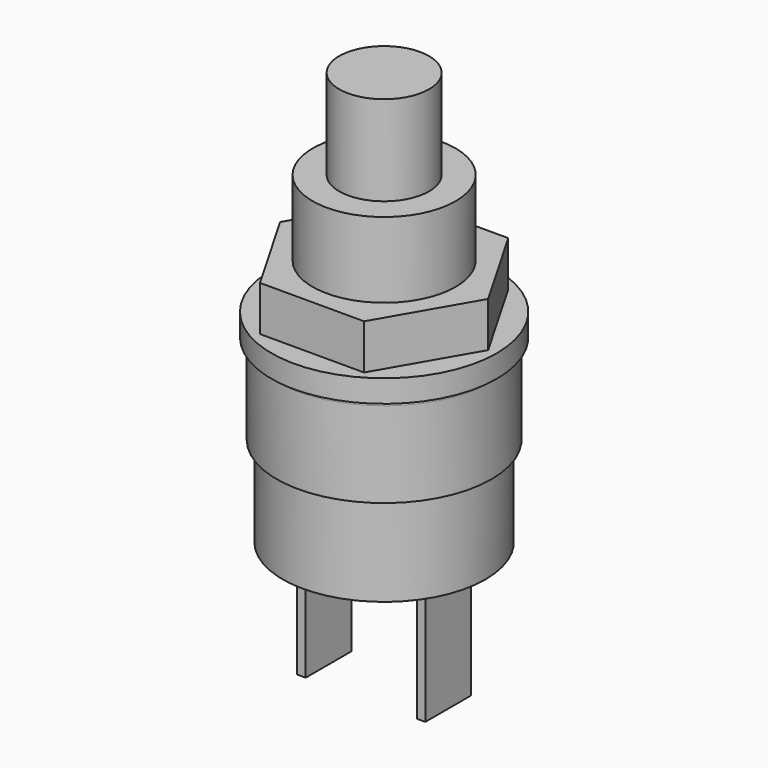
from build123d import *

# Parameters (mm, degrees)
F0_R      = 1.995
F1_DEPTH  = 14.34
F0_R_2    = 3.175
F2_DEPTH  = 10.35
F0_R_3    = 4.765
F0_R_4    = 4.5
F3_DEPTH  = 4
F4_DEPTH  = 4
F5_W      = 0.38
F5_H      = 2.54
F6_DEPTH  = 5.59
F7_R      = 0.2
F8_R      = 5
F8_R_2    = 3.4
F9_DEPTH  = 1
F10_R     = 2.75
F11_DEPTH = 2


with BuildPart() as f1:
    # F0 (on Top) → F1 (new body)
    with BuildSketch(Plane.XY):
        Circle(F0_R)
    extrude(amount=F1_DEPTH)


with BuildPart() as f2:
    # F0 (on Top) → F2 (new body)
    with BuildSketch(Plane.XY):
        Circle(F0_R_2)
        Circle(F0_R, mode=Mode.SUBTRACT)
        Circle(F0_R)
    extrude(amount=F2_DEPTH)

    # F0 (on Top) → F3 (join)
    with BuildSketch(Plane.XY):
        Circle(F0_R_3)
        Circle(F0_R_4, mode=Mode.SUBTRACT)
        Circle(F0_R_4)
        Circle(F0_R_2, mode=Mode.SUBTRACT)
        Circle(F0_R_2)
        Circle(F0_R, mode=Mode.SUBTRACT)
        Circle(F0_R)
    extrude(amount=F3_DEPTH)

    # F0 (on Top) → F4 (join)
    with BuildSketch(Plane.XY):
        Circle(F0_R_4)
        Circle(F0_R_2, mode=Mode.SUBTRACT)
        Circle(F0_R_2)
        Circle(F0_R, mode=Mode.SUBTRACT)
        Circle(F0_R)
    extrude(amount=-F4_DEPTH)

    # F5 (on face) → F6 (join)
    with BuildSketch(Plane(origin=(0, 0, -4), x_dir=(1, 0, 0), z_dir=(0, 0, -1))):
        with Locations((-2.655, 0)):
            Rectangle(F5_W, F5_H)
        with Locations((2.655, 0)):
            Rectangle(F5_W, F5_H)
    extrude(amount=F6_DEPTH)

    # F7
    f7_edges = [f2.edges().sort_by_distance(p)[0] for p in [
        (-4.765, 0, 4),
    ]]
    fillet(f7_edges, radius=F7_R)


with BuildPart() as f9:
    # F8 (on face) → F9 (new body)
    with BuildSketch(Plane.XY.offset(4)):
        Circle(F8_R)
        Circle(F8_R_2, mode=Mode.SUBTRACT)
    extrude(amount=F9_DEPTH)


with BuildPart() as f11:
    # F10 (on face) → F11 (new body)
    with BuildSketch(Plane.XY.offset(5)):
        Polygon((2.3094010768, 4), (-2.3094010768, 4), (-4.6188021535, 0), (-2.3094010768, -4), (2.3094010768, -4), (4.6188021535, 0), align=None)
        Circle(F10_R, mode=Mode.SUBTRACT)
    extrude(amount=F11_DEPTH)


solid = Compound([f1.part, f2.part, f9.part, f11.part])
